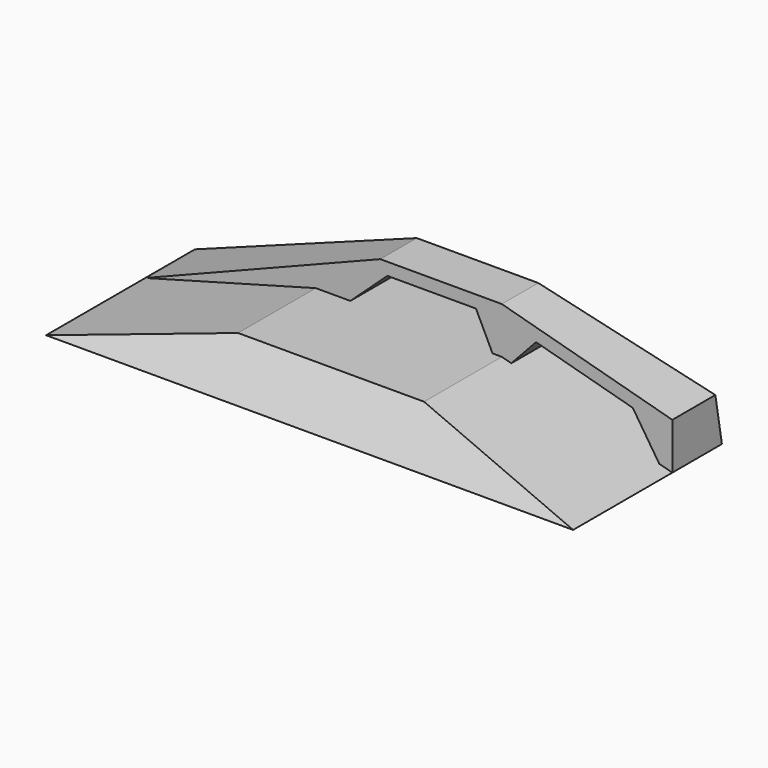
from build123d import *

# Parameters (mm, degrees)
F2_DEPTH = 800
F3_DEPTH = 2400
F5_DEPTH = 6800.001


# Not quite as in the source:
# - a feature names something its author has since deleted; it is built from what else it names


with BuildPart() as f2:
    # F1 (on Front) → F2 (new body)
    with BuildSketch(Plane.XZ):
        Polygon((3231.4479728419, 45.9687346795), (3400, 0), (3400, 600), (1200, 1200), (-367.7977621555, 1200), (-3400, 0), (-1200, 600), (-754.085123539, 600), (-276.6310870647, 1039.9327278137), (866.5578365326, 1039.9327278137), (1168.6351299286, 1039.9327278137), (1641.5758518072, 910.9488945741), (2889.8836052394, 570.5013254562), align=None)
        Polygon((1200, 600), (1322.2261014351, 566.6656086995), (1641.5758518072, 910.9488945741), (1168.6351299286, 1039.9327278137), (866.5578365326, 1039.9327278137), (1080.6080102921, 600), align=None)
    extrude(amount=F2_DEPTH)

    # F1 (on Front) → F3 (join)
    with BuildSketch(Plane.XZ):
        Polygon((-3400, 0), (3400, 0), (3231.4479728419, 45.9687346795), (1322.2261014351, 566.6656086995), (1200, 600), (1080.6080102921, 600), (-754.085123539, 600), (-1200, 600), align=None)
    extrude(amount=F3_DEPTH)

    # F4 (on face) → F5 (cut, through all)
    with BuildSketch(Plane.YZ.offset(3400)):
        Polygon((0, 600), (0, 1200), (-211.5923768502, 1200), (-105.7961884251, 600), align=None)
        Polygon((0, 0), (0, 600), (-105.7961884251, 600), align=None)
        Polygon((-2400, 600), (-2400, 0), (-2053.5898384862, 600), align=None)
    extrude(amount=-F5_DEPTH, mode=Mode.SUBTRACT)


solid = f2.part
